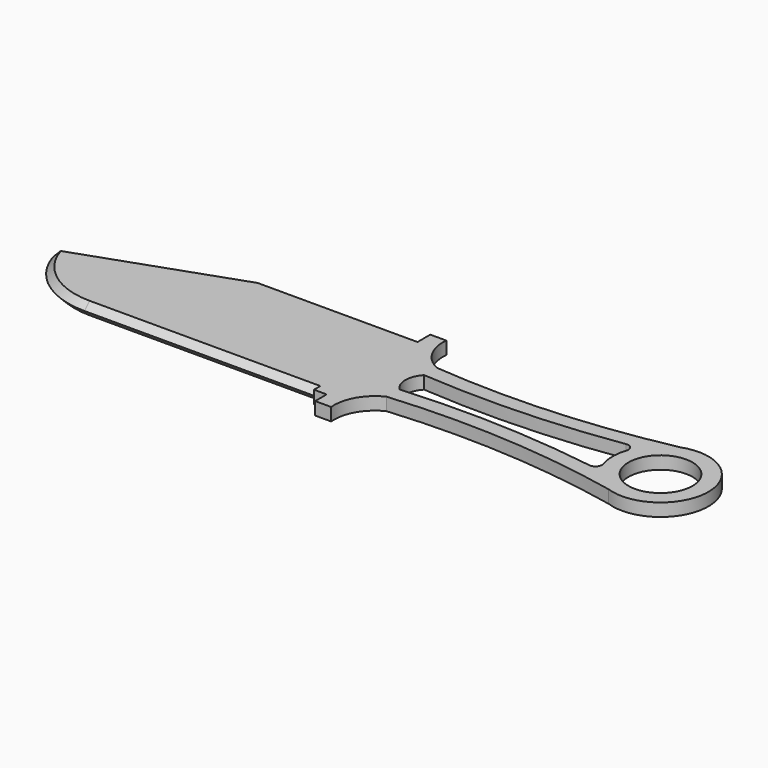
from build123d import *

# Parameters (mm, degrees)
F0_R     = 10
F1_DEPTH = 4
F2_R     = 2
F3_W     = 4
F3_H     = 4
F4_DEPTH = 0.5
F5_SIZE  = 1.99999


# Not quite as in the source:
# - a fillet or chamfer is up to 0.001 mm smaller than in the source, because OpenCascade refuses the exact size


with BuildPart() as f1:
    # F0 (on Top) → F1 (new body)
    with BuildSketch(Plane.XY):
        with BuildLine():
            Line((50, 22.5), (50, 17.5))
            Line((50, 17.5), (0, 17.5))
            Line((0, 17.5), (-50, 0))
            ThreePointArc((-50, 0), (-40.9417194223, -12.6556443707), (-26.1515199646, -17.5))
            Line((-26.1515199646, -17.5), (50, -17.5))
            Line((50, -17.5), (50, -22.5))
            Line((50, -22.5), (55, -22.5))
            ThreePointArc((55, -22.5), (56.5936558821, -15.0125045804), (62.1990375221, -9.7988663689))
            ThreePointArc((62.1990375221, -9.7988663689), (98.7587484272, -9.3015269429), (135, -14.1421356237))
            ThreePointArc((135, -14.1421356237), (155, 0), (135, 14.1421356237))
            ThreePointArc((135, 14.1421356237), (98.7587484272, 9.3015269429), (62.1990375221, 9.7988663689))
            ThreePointArc((62.1990375221, 9.7988663689), (56.5936558821, 15.0125045804), (55, 22.5))
            Line((55, 22.5), (50, 22.5))
        make_face()
        with BuildLine():
            ThreePointArc((62.1990375221, -4.8343795659), (60.2509894701, 0), (62.1990375221, 4.8343795659))
            ThreePointArc((62.1990375221, 4.8343795659), (94.7590329876, 4.3577585856), (127.1470964452, 7.7332315503))
            ThreePointArc((127.1470964452, 7.7332315503), (125, 0), (127.1470964452, -7.7332315503))
            ThreePointArc((127.1470964452, -7.7332315503), (94.7590329876, -4.3577585856), (62.1990375221, -4.8343795659))
        make_face(mode=Mode.SUBTRACT)
        with Locations((140, 0)):
            Circle(F0_R, mode=Mode.SUBTRACT)
    extrude(amount=F1_DEPTH)

    # F2
    f2_edges = [f1.edges().sort_by_distance(p)[0] for p in [
        (127.147096, 7.733232, 2),
        (127.147096, -7.733232, 2),
    ]]
    fillet(f2_edges, radius=F2_R)

    # F3 (on face) → F4 (join)
    with BuildSketch(Plane.XZ.offset(17.5)):
        with Locations((48, 2)):
            Rectangle(F3_W, F3_H)
    extrude(amount=F4_DEPTH)

    # F5 (size 2 in the source; OpenCascade refuses exactly that, so slightly less here)
    f5_edges = [f1.edges().sort_by_distance(p)[0] for p in [
        (9.92424, -17.5, 4),
        (9.92424, -17.5, 0),
    ]]
    chamfer(f5_edges, length=F5_SIZE)


solid = f1.part
